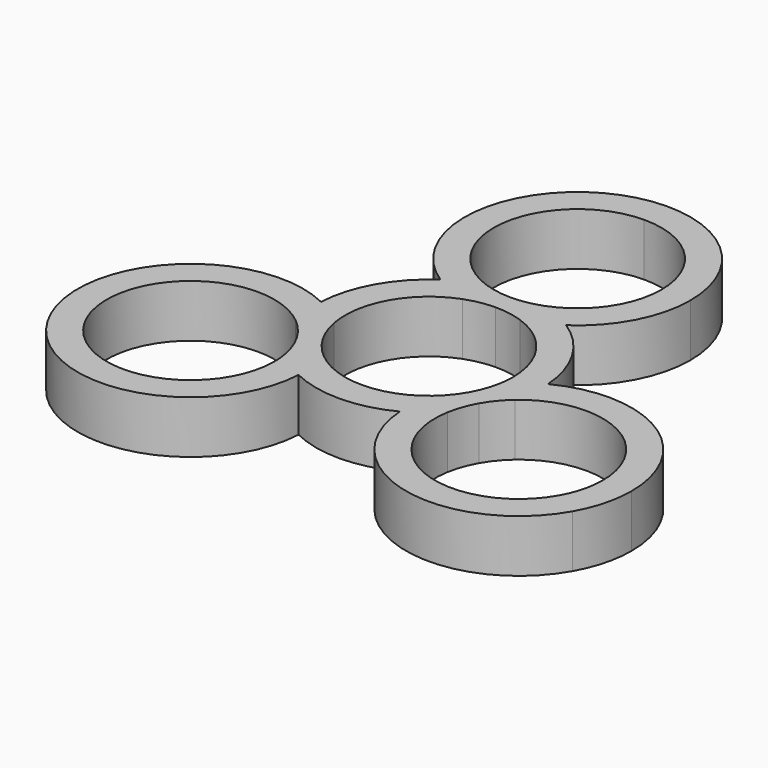
from build123d import *

# Parameters (mm, degrees)
F1_DEPTH = 7


with BuildPart() as f1:
    # F0 (on Top) → F1 (new body)
    with BuildSketch(Plane.XY):
        with BuildLine():
            ThreePointArc((-3.8906200654, 10.4491901843), (-2.0298332845, 10.9636798949), (-0.1081914722, 11.1494750821))
            Line((-0.1081914722, 11.1494750821), (-0.1343903041, 13.8493479719))
            ThreePointArc((-0.1343903041, 13.8493479719), (-2.0592757302, 13.9978175054), (-3.9296961082, 14.4761005971))
            ThreePointArc((-3.9296961082, 14.4761005971), (-6.2562113602, 13.6330414588), (-8.4124625152, 12.4189562537))
            ThreePointArc((-8.4124625152, 12.4189562537), (-6.2330573108, 11.2469430781), (-3.8906200654, 10.4491901843))
        make_face()
        with BuildLine():
            Line((-0.1343903041, 13.8493479719), (-0.1081914722, 11.1494750821))
            ThreePointArc((-0.1081914722, 11.1494750821), (1.8166939539, 11.0010055485), (3.6871143319, 10.5227224568))
            ThreePointArc((3.6871143319, 10.5227224568), (6.0136295839, 11.3657815952), (8.1698807389, 12.5798668003))
            ThreePointArc((8.1698807389, 12.5798668003), (5.9904755345, 13.7518799759), (3.648038289, 14.5496328697))
            ThreePointArc((3.648038289, 14.5496328697), (1.7872515082, 14.0351431591), (-0.1343903041, 13.8493479719))
        make_face()
        with BuildLine():
            ThreePointArc((-10.9565021305, -2.0682265504), (-9.709824396, 5.4810409776), (-3.8906200654, 10.4491901843))
            ThreePointArc((-3.8906200654, 10.4491901843), (-6.2330573108, 11.2469430781), (-8.4124625152, 12.4189562537))
            ThreePointArc((-8.4124625152, 12.4189562537), (-13.0625440306, 7.3735977277), (-14.9794245947, 0.7853908656))
            ThreePointArc((-14.9794245947, 0.7853908656), (-12.8498703872, -0.474934809), (-10.9565021305, -2.0682265504))
        make_face()
        with BuildLine():
            ThreePointArc((8.1698807389, 12.5798668003), (6.0136295839, 11.3657815952), (3.6871143319, 10.5227224568))
            ThreePointArc((3.6871143319, 10.5227224568), (9.0948838585, 6.4502393444), (11.15, 0))
            ThreePointArc((11.15, 0), (11.1110756032, -0.930859248), (10.9945741812, -1.8552192791))
            ThreePointArc((10.9945741812, -1.8552192791), (12.8566670759, -0.2254855646), (14.9613628618, 1.0759281197))
            ThreePointArc((14.9613628618, 1.0759281197), (12.9169949647, 7.6256961047), (8.1698807389, 12.5798668003))
        make_face()
        with BuildLine():
            ThreePointArc((10.9945741812, -1.8552192791), (10.5097419502, -3.7239527576), (9.709824396, -5.4810409776))
            Line((9.709824396, -5.4810409776), (12.0610823215, -6.8082885686))
            ThreePointArc((12.0610823215, -6.8082885686), (13.1521034224, -5.2155236569), (14.5015189189, -3.8348336397))
            ThreePointArc((14.5015189189, -3.8348336397), (14.87485771, -1.933548062), (15, 0))
            ThreePointArc((15, 0), (14.9903376034, 0.538310818), (14.9613628618, 1.0759281197))
            ThreePointArc((14.9613628618, 1.0759281197), (12.8566670759, -0.2254855646), (10.9945741812, -1.8552192791))
        make_face()
        with BuildLine():
            Line((12.0610823215, -6.8082885686), (9.709824396, -5.4810409776))
            ThreePointArc((9.709824396, -5.4810409776), (8.6188032952, -7.0738058892), (7.2693877987, -8.4544959065))
            ThreePointArc((7.2693877987, -8.4544959065), (6.8362408033, -10.8908467862), (6.8095438558, -13.3652576659))
            ThreePointArc((6.8095438558, -13.3652576659), (8.9142396416, -12.0638439816), (10.7763325364, -10.4341102671))
            ThreePointArc((10.7763325364, -10.4341102671), (11.2611647674, -8.5653767885), (12.0610823215, -6.8082885686))
        make_face()
        with BuildLine():
            ThreePointArc((6.8095438558, -13.3652576659), (6.8362408033, -10.8908467862), (7.2693877987, -8.4544959065))
            ThreePointArc((7.2693877987, -8.4544959065), (0.1081914722, -11.1494750821), (-7.1039541159, -8.5939709052))
            ThreePointArc((-7.1039541159, -8.5939709052), (-6.6729292484, -10.6317016968), (-6.5283249412, -12.7094935078))
            ThreePointArc((-6.5283249412, -12.7094935078), (-6.5334696748, -13.1023236743), (-6.5489003466, -13.4948843734))
            ThreePointArc((-6.5489003466, -13.4948843734), (0.1455490658, -14.9992938324), (6.8095438558, -13.3652576659))
        make_face()
        with BuildLine():
            ThreePointArc((-7.1039541159, -8.5939709052), (-8.4799086657, -7.2397271373), (-9.6016329238, -5.6684341045))
            Line((-9.6016329238, -5.6684341045), (-11.9266920175, -7.0410594033))
            ThreePointArc((-11.9266920175, -7.0410594033), (-11.0928276921, -8.7822938485), (-10.5718228107, -10.6412669574))
            ThreePointArc((-10.5718228107, -10.6412669574), (-8.678454554, -12.2345586988), (-6.5489003466, -13.4948843734))
            ThreePointArc((-6.5489003466, -13.4948843734), (-6.5334696748, -13.1023236743), (-6.5283249412, -12.7094935078))
            ThreePointArc((-6.5283249412, -12.7094935078), (-6.6729292484, -10.6317016968), (-7.1039541159, -8.5939709052))
        make_face()
        with BuildLine():
            Line((-11.9266920175, -7.0410594033), (-9.6016329238, -5.6684341045))
            ThreePointArc((-9.6016329238, -5.6684341045), (-10.4354972491, -3.9271996593), (-10.9565021305, -2.0682265504))
            ThreePointArc((-10.9565021305, -2.0682265504), (-12.8498703872, -0.474934809), (-14.9794245947, 0.7853908656))
            ThreePointArc((-14.9794245947, 0.7853908656), (-14.9047151761, -1.6880359943), (-14.4243708254, -4.1155226026))
            ThreePointArc((-14.4243708254, -4.1155226026), (-13.0484162756, -5.4697663705), (-11.9266920175, -7.0410594033))
        make_face()
        with BuildLine():
            ThreePointArc((-0.3881308421, 39.9981168863), (-14.6453286848, 29.1893935987), (-8.4124625152, 12.4189562537))
            ThreePointArc((-8.4124625152, 12.4189562537), (-6.2562113602, 13.6330414588), (-3.9296961082, 14.4761005971))
            ThreePointArc((-3.9296961082, 14.4761005971), (-11.2435873248, 26.8155170078), (-0.3507732486, 36.148298136))
            Line((-0.3507732486, 36.148298136), (-0.3881308421, 39.9981168863))
        make_face()
        with BuildLine():
            ThreePointArc((3.648038289, 14.5496328697), (5.9904755345, 13.7518799759), (8.1698807389, 12.5798668003))
            ThreePointArc((8.1698807389, 12.5798668003), (13.0085868085, 17.9698450958), (14.7574182237, 24.9988230539))
            ThreePointArc((14.7574182237, 24.9988230539), (10.3124351354, 35.6567599084), (-0.3881308421, 39.9981168863))
            Line((-0.3881308421, 39.9981168863), (-0.3507732486, 36.148298136))
            ThreePointArc((-0.3507732486, 36.148298136), (7.603314128, 32.9212227824), (10.9074182237, 24.9988230539))
            ThreePointArc((10.9074182237, 24.9988230539), (8.9144623354, 18.6371374962), (3.648038289, 14.5496328697))
        make_face()
        with BuildLine():
            ThreePointArc((36.7709067176, -12.2893295462), (29.6085352544, 0.5001809573), (14.9613628618, 1.0759281197))
            ThreePointArc((14.9613628618, 1.0759281197), (14.9903376034, 0.538310818), (15, 0))
            ThreePointArc((15, 0), (14.87485771, -1.933548062), (14.5015189189, -3.8348336397))
            ThreePointArc((14.5015189189, -3.8348336397), (26.4221875114, -2.1558164842), (32.9209067176, -12.2893295462))
            ThreePointArc((32.9209067176, -12.2893295462), (32.5548540936, -15.1228748506), (31.4807311136, -17.7703705237))
            Line((31.4807311136, -17.7703705237), (34.8334507481, -19.6629272739))
            ThreePointArc((34.8334507481, -19.6629272739), (36.2784592413, -16.1012739018), (36.7709067176, -12.2893295462))
        make_face()
        with BuildLine():
            ThreePointArc((10.7763325364, -10.4341102671), (8.9142396416, -12.0638439816), (6.8095438558, -13.3652576659))
            ThreePointArc((6.8095438558, -13.3652576659), (18.4820560276, -26.9243376138), (34.8334507481, -19.6629272739))
            Line((34.8334507481, -19.6629272739), (31.4807311136, -17.7703705237))
            ThreePointArc((31.4807311136, -17.7703705237), (18.04695396, -22.7990714963), (10.7763325364, -10.4341102671))
        make_face()
        with BuildLine():
            ThreePointArc((-14.4243708254, -4.1155226026), (-14.9047151761, -1.6880359943), (-14.9794245947, 0.7853908656))
            ThreePointArc((-14.9794245947, 0.7853908656), (-32.5581883674, -2.5437612272), (-34.445319906, -20.3351896124))
            Line((-34.445319906, -20.3351896124), (-31.129957865, -18.3779276122))
            ThreePointArc((-31.129957865, -18.3779276122), (-28.7680520785, -4.2295848421), (-14.4243708254, -4.1155226026))
        make_face()
        with BuildLine():
            ThreePointArc((-34.445319906, -20.3351896124), (-17.9560920351, -27.2779234872), (-6.5489003466, -13.4948843734))
            ThreePointArc((-6.5489003466, -13.4948843734), (-8.678454554, -12.2345586988), (-10.5718228107, -10.6412669574))
            ThreePointArc((-10.5718228107, -10.6412669574), (-10.4268048031, -11.6708643043), (-10.3783249412, -12.7094935078))
            ThreePointArc((-10.3783249412, -12.7094935078), (-18.5902734696, -23.4654385406), (-31.129957865, -18.3779276122))
            Line((-31.129957865, -18.3779276122), (-34.445319906, -20.3351896124))
        make_face()
    extrude(amount=F1_DEPTH)


solid = f1.part
